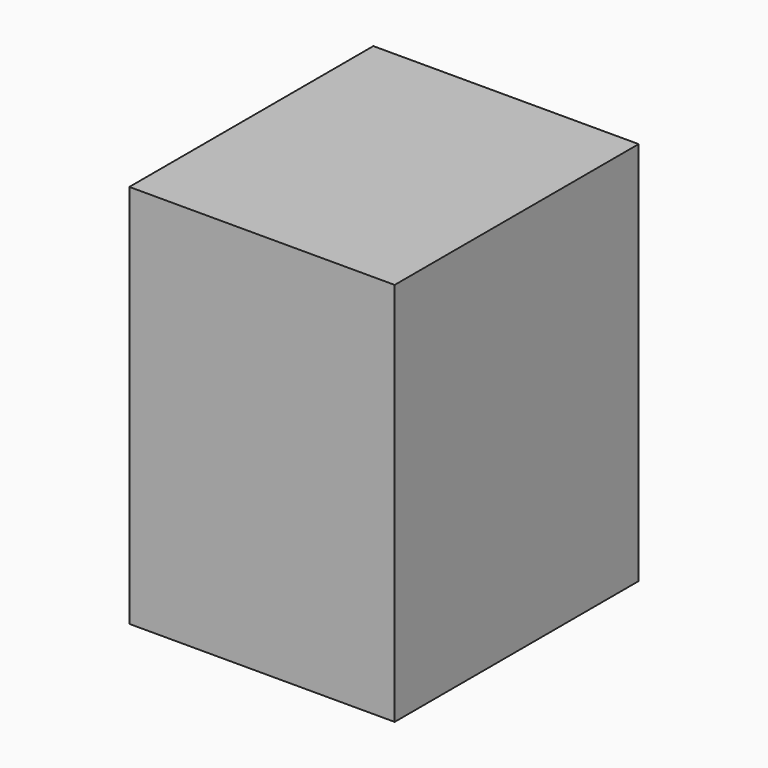
from build123d import *

# Parameters (mm, degrees)
F0_W     = 106.3328497112
F0_H     = 191.0245120525
F1_DEPTH = 25.4
F5_DEPTH = 100.6231699139
F2_DEPTH = 25.4
F3_DEPTH = 25.4


# Not quite as in the source:
# - the program builds the solid bodies; features that only make, move or delete a surface that nothing else refers to are left out


with BuildPart() as f1:
    # F0 (on Front) → F1 (new body)
    with BuildSketch(Plane.XZ):
        with Locations((-6.1664935201, -12.889765203)):
            Rectangle(F0_W, F0_H)
    extrude(amount=F1_DEPTH)

    # F5 (add): a face of the model
    f5_faces = [f1.faces().sort_by_distance(p)[0] for p in [
        (-6.1664935201, -25.4, -12.889765203),
    ]]
    extrude(f5_faces, amount=F5_DEPTH)

    # F2 (add): a face of the model
    f2_faces = [f1.faces().sort_by_distance(p)[0] for p in [
        (46.9999313354, -63.0115849569, -12.889765203),
    ]]
    extrude(f2_faces, amount=F2_DEPTH)

    # F3 (add): a face of the model
    f3_faces = [f1.faces().sort_by_distance(p)[0] for p in [
        (6.5335064799, 0, -12.889765203),
    ]]
    extrude(f3_faces, amount=F3_DEPTH)


solid = f1.part
